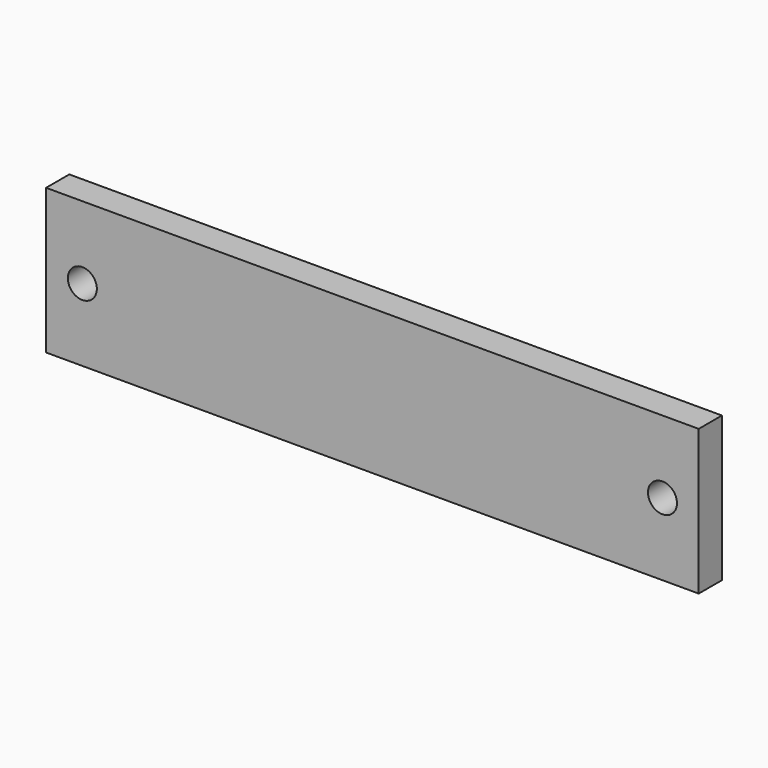
from build123d import *

# Parameters (mm, degrees)
F0_W     = 450
F0_H     = 100
F1_DEPTH = 10
F2_R     = 10
F3_DEPTH = 20.001


# Not quite as in the source:
# - a pattern or mirror of a feature is missing from the dataset's text; its kind, count and spacing are read off the source's solid


with BuildPart() as f1:
    # F0 (on Front) → F1 (new body, symmetric)
    with BuildSketch(Plane.XZ):
        Rectangle(F0_W, F0_H)
    extrude(amount=F1_DEPTH, both=True)

    # F2 (on face) → F3 (cut, through all)
    with BuildSketch(Plane.XZ.offset(10)):
        with Locations((-200, 0)):
            Circle(F2_R)
    f3 = extrude(amount=-F3_DEPTH, mode=Mode.SUBTRACT)

    # F3_copies: F3 across plane
    add(f3.mirror(Plane(origin=(0, 0, 0), x_dir=(0, 0, 1), z_dir=(1, 0, 0))), mode=Mode.SUBTRACT)


solid = f1.part
